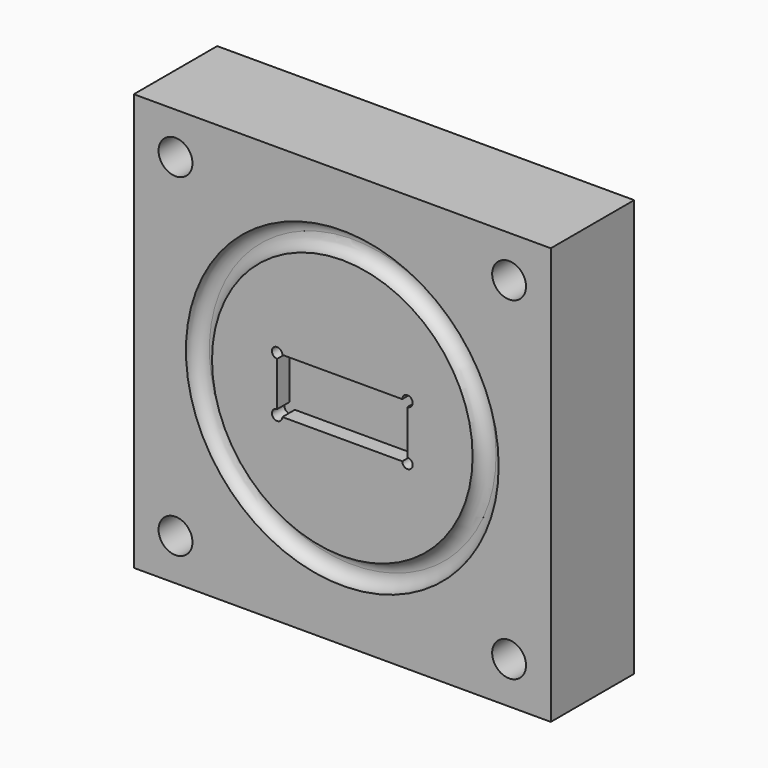
from build123d import *

# Parameters (mm, degrees)
F1_W     = 80
F1_H     = 80
F2_DEPTH = 20
F4_R     = 3.25
F5_DEPTH = 20.001
F4_R_2   = 30
F4_R_3   = 25
F6_DEPTH = 2.5
F7_DEPTH = 3
F8_R     = 2.49999
F9_R     = 2.49999


# Not quite as in the source:
# - a fillet or chamfer is up to 0.001 mm smaller than in the source, because OpenCascade refuses the exact size


with BuildPart() as f2:
    # F1 (on Front) → F2 (new body)
    with BuildSketch(Plane.XZ):
        with Locations((40, 40)):
            Rectangle(F1_W, F1_H)
    extrude(amount=F2_DEPTH)

    # F4 (on face) → F5 (cut, through all)
    with BuildSketch(Plane.XZ.offset(20)):
        with Locations((72, 8)):
            Circle(F4_R)
        with Locations((8, 8)):
            Circle(F4_R)
        with Locations((8, 72)):
            Circle(F4_R)
        with Locations((72, 72)):
            Circle(F4_R)
    extrude(amount=-F5_DEPTH, mode=Mode.SUBTRACT)

    # F4 (on face) → F6 (cut)
    with BuildSketch(Plane.XZ.offset(20)):
        with Locations((40, 40)):
            Circle(F4_R_2)
        with Locations((40, 40)):
            Circle(F4_R_3, mode=Mode.SUBTRACT)
    extrude(amount=-F6_DEPTH, mode=Mode.SUBTRACT)

    # F4 (on face) → F7 (cut)
    with BuildSketch(Plane.XZ.offset(20)):
        with BuildLine():
            Line((28.5, 45.25), (27.5, 45.25))
            Line((27.5, 45.25), (27.5, 44.25))
            ThreePointArc((27.5, 44.25), (28.2071067812, 44.5428932188), (28.5, 45.25))
        make_face()
        with BuildLine():
            Line((51.5, 45.25), (28.5, 45.25))
            ThreePointArc((28.5, 45.25), (28.2071067812, 44.5428932188), (27.5, 44.25))
            Line((27.5, 44.25), (27.5, 40))
            Line((27.5, 40), (52.5, 40))
            Line((52.5, 40), (52.5, 44.25))
            ThreePointArc((52.5, 44.25), (51.7928932188, 44.5428932188), (51.5, 45.25))
        make_face()
        with BuildLine():
            Line((52.5, 45.25), (51.5, 45.25))
            ThreePointArc((51.5, 45.25), (51.7928932188, 44.5428932188), (52.5, 44.25))
            Line((52.5, 44.25), (52.5, 45.25))
        make_face()
        with BuildLine():
            ThreePointArc((28.5, 34.75), (28.2071067812, 35.4571067812), (27.5, 35.75))
            Line((27.5, 35.75), (27.5, 34.75))
            Line((27.5, 34.75), (28.5, 34.75))
        make_face()
        with BuildLine():
            Line((52.5, 40), (27.5, 40))
            Line((27.5, 40), (27.5, 35.75))
            ThreePointArc((27.5, 35.75), (28.2071067812, 35.4571067812), (28.5, 34.75))
            Line((28.5, 34.75), (51.5, 34.75))
            ThreePointArc((51.5, 34.75), (51.7928932188, 35.4571067812), (52.5, 35.75))
            Line((52.5, 35.75), (52.5, 40))
        make_face()
        with BuildLine():
            Line((52.5, 34.75), (52.5, 35.75))
            ThreePointArc((52.5, 35.75), (51.7928932188, 35.4571067812), (51.5, 34.75))
            Line((51.5, 34.75), (52.5, 34.75))
        make_face()
        with BuildLine():
            Line((27.5, 34.75), (27.5, 35.75))
            ThreePointArc((27.5, 35.75), (26.7928932188, 34.0428932188), (28.5, 34.75))
            Line((28.5, 34.75), (27.5, 34.75))
        make_face()
        with BuildLine():
            ThreePointArc((53.5, 34.75), (53.2071067812, 35.4571067812), (52.5, 35.75))
            Line((52.5, 35.75), (52.5, 34.75))
            Line((52.5, 34.75), (51.5, 34.75))
            ThreePointArc((51.5, 34.75), (52.5, 33.75), (53.5, 34.75))
        make_face()
        with BuildLine():
            ThreePointArc((53.5, 45.25), (52.5, 46.25), (51.5, 45.25))
            Line((51.5, 45.25), (52.5, 45.25))
            Line((52.5, 45.25), (52.5, 44.25))
            ThreePointArc((52.5, 44.25), (53.2071067812, 44.5428932188), (53.5, 45.25))
        make_face()
        with BuildLine():
            Line((27.5, 44.25), (27.5, 45.25))
            Line((27.5, 45.25), (28.5, 45.25))
            ThreePointArc((28.5, 45.25), (26.7928932188, 45.9571067812), (27.5, 44.25))
        make_face()
    extrude(amount=-F7_DEPTH, mode=Mode.SUBTRACT)

    # F8 (radius 2.5 in the source; OpenCascade refuses exactly that, so slightly less here)
    f8_edges = [f2.edges().sort_by_distance(p)[0] for p in [
        (15, -17.5, 40),
    ]]
    fillet(f8_edges, radius=F8_R)

    # F9 (radius 2.5 in the source; OpenCascade refuses exactly that, so slightly less here)
    f9_edges = [f2.edges().sort_by_distance(p)[0] for p in [
        (10, -17.5, 40),
    ]]
    fillet(f9_edges, radius=F9_R)


solid = f2.part
